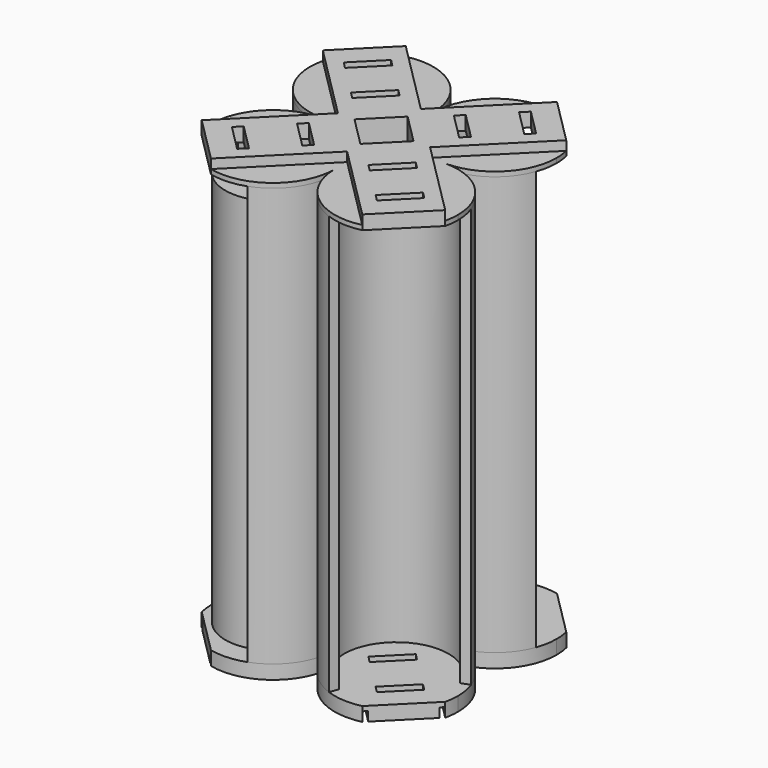
from build123d import *
from build123d import SkipClean  # not in build123d's __all__

# Parameters (mm, degrees)
F1_DEPTH  = 22.5
F2_R      = 5.125
F3_DEPTH  = 43
F4_R      = 1.75
F5_DEPTH  = 2
F6_R      = 5.125
F6_R_2    = 3
F7_DEPTH  = 0.5
F9_DEPTH  = 0.5
F11_DEPTH = 1.5
F13_DEPTH = 1
F14_DEPTH = 47.001
F16_DEPTH = 1


# Not quite as in the source:
# - after a boolean that leaves OpenCascade's solid faulty, fix() repairs it


with BuildPart() as f1:
    # F0 (on Top) → F1 (new body, symmetric)
    with BuildSketch(Plane.XY):
        with BuildLine():
            ThreePointArc((-4.7011366938, 11.9107709919), (-2.0172697509, 9.8513674545), (-1, 6.625))
            ThreePointArc((-1, 6.625), (-5.6482290006, 1.0854563893), (-11.9107709919, 4.7011366938))
            Line((-11.9107709919, 4.7011366938), (-12.8504636127, 4.3591165505))
            ThreePointArc((-12.8504636127, 4.3591165505), (-10.4249438908, 1.1981177066), (-6.625, 0))
            ThreePointArc((-6.625, 0), (-10.4249438908, -1.1981177066), (-12.8504636127, -4.3591165505))
            Line((-12.8504636127, -4.3591165505), (-11.9107709919, -4.7011366938))
            ThreePointArc((-11.9107709919, -4.7011366938), (-5.6482290006, -1.0854563893), (-1, -6.625))
            ThreePointArc((-1, -6.625), (-2.0172697509, -9.8513674545), (-4.7011366938, -11.9107709919))
            Line((-4.7011366938, -11.9107709919), (-4.3591165505, -12.8504636127))
            ThreePointArc((-4.3591165505, -12.8504636127), (-1.1981177066, -10.4249438908), (0, -6.625))
            ThreePointArc((0, -6.625), (1.1981177066, -10.4249438908), (4.3591165505, -12.8504636127))
            Line((4.3591165505, -12.8504636127), (4.7011366938, -11.9107709919))
            ThreePointArc((4.7011366938, -11.9107709919), (2.6475243558, -2.6475243558), (11.9107709919, -4.7011366938))
            Line((11.9107709919, -4.7011366938), (12.8504636127, -4.3591165505))
            ThreePointArc((12.8504636127, -4.3591165505), (10.4249438908, -1.1981177066), (6.625, 0))
            ThreePointArc((6.625, 0), (10.4249438908, 1.1981177066), (12.8504636127, 4.3591165505))
            Line((12.8504636127, 4.3591165505), (11.9107709919, 4.7011366938))
            ThreePointArc((11.9107709919, 4.7011366938), (2.6475243558, 2.6475243558), (4.7011366938, 11.9107709919))
            Line((4.7011366938, 11.9107709919), (4.3591165505, 12.8504636127))
            ThreePointArc((4.3591165505, 12.8504636127), (1.1981177066, 10.4249438908), (0, 6.625))
            ThreePointArc((0, 6.625), (-1.1981177066, 10.4249438908), (-4.3591165505, 12.8504636127))
            Line((-4.3591165505, 12.8504636127), (-4.7011366938, 11.9107709919))
        make_face()
        Polygon((0, -3.1737283681), (-3.1737283681, 0), (0, 3.1737283681), (3.1737283681, 0), align=None, mode=Mode.SUBTRACT)
    extrude(amount=F1_DEPTH, both=True)

    # F8 (on face) → F9 (join)
    with BuildSketch(Plane.XY.offset(22.5)):
        with BuildLine():
            ThreePointArc((-6.625, 0), (-11.3095824254, -11.3095824254), (0, -6.625))
            ThreePointArc((0, -6.625), (-1.9404175746, -1.9404175746), (-6.625, 0))
        make_face()
        Polygon((-10.3373106012, -7.5088834765), (-9.63020382, -6.8017766953), (-6.8017766953, -9.63020382), (-7.5088834765, -10.3373106012), align=None, mode=Mode.SUBTRACT)
        Polygon((-2.9126893988, -5.7411165235), (-3.61979618, -6.4482233047), (-6.4482233047, -3.61979618), (-5.7411165235, -2.9126893988), align=None, mode=Mode.SUBTRACT)
        with BuildLine():
            ThreePointArc((6.6250000363, 0), (1.9404175875, -1.9404175618), (0, -6.625))
            ThreePointArc((0, -6.625), (6.625, -13.25), (13.25, -6.625))
            ThreePointArc((13.25, -6.625), (11.3095824382, -1.9404175875), (6.6250000363, 0))
        make_face()
        Polygon((7.5088834765, -10.3373106012), (6.8017766953, -9.63020382), (9.63020382, -6.8017766953), (10.3373106012, -7.5088834765), align=None, mode=Mode.SUBTRACT)
        Polygon((2.9126893988, -5.7411165235), (5.7411165235, -2.9126893988), (6.4482233047, -3.61979618), (3.61979618, -6.4482233047), align=None, mode=Mode.SUBTRACT)
        with BuildLine():
            ThreePointArc((-6.625, 0), (-1.9404175746, -1.9404175746), (0, -6.625))
            ThreePointArc((0, -6.625), (1.9404175875, -1.9404175618), (6.6250000363, 0))
            ThreePointArc((6.6250000363, 0), (1.9404175875, 1.9404175618), (0, 6.625))
            ThreePointArc((0, 6.625), (-1.9404175746, 1.9404175746), (-6.625, 0))
        make_face()
        Polygon((0, -3.1737283681), (-3.1737283681, 0), (0, 3.1737283681), (3.1737283681, 0), align=None, mode=Mode.SUBTRACT)
        with BuildLine():
            ThreePointArc((0, 6.625), (-11.3095824254, 11.3095824254), (-6.625, 0))
            ThreePointArc((-6.625, 0), (-1.9404175746, 1.9404175746), (0, 6.625))
        make_face()
        Polygon((-2.9126893988, 5.7411165235), (-5.7411165235, 2.9126893988), (-6.4482233047, 3.61979618), (-3.61979618, 6.4482233047), align=None, mode=Mode.SUBTRACT)
        Polygon((-7.5088834765, 10.3373106012), (-6.8017766953, 9.63020382), (-9.63020382, 6.8017766953), (-10.3373106012, 7.5088834765), align=None, mode=Mode.SUBTRACT)
        with BuildLine():
            ThreePointArc((0, 6.625), (1.9404175875, 1.9404175618), (6.6250000363, 0))
            ThreePointArc((6.6250000363, 0), (11.3095824382, 1.9404175875), (13.25, 6.625))
            ThreePointArc((13.25, 6.625), (6.625, 13.25), (0, 6.625))
        make_face()
        Polygon((6.4482233047, 3.61979618), (5.7411165235, 2.9126893988), (2.9126893988, 5.7411165235), (3.61979618, 6.4482233047), align=None, mode=Mode.SUBTRACT)
        Polygon((9.63020382, 6.8017766953), (6.8017766953, 9.63020382), (7.5088834765, 10.3373106012), (10.3373106012, 7.5088834765), align=None, mode=Mode.SUBTRACT)
    with SkipClean():  # cleaning this boolean's faces spoils the solid; the shape is the same uncleaned
        extrude(amount=F9_DEPTH)

    # F10 (on face) → F11 (join)
    with BuildSketch(Plane(origin=(0, 0, -22.5), x_dir=(1, 0, 0), z_dir=(0, 0, -1))):
        with BuildLine():
            ThreePointArc((-6.625, 0), (-11.3095824254, -11.3095824254), (0, -6.625))
            ThreePointArc((0, -6.625), (-1.9404175746, -1.9404175746), (-6.625, 0))
        make_face()
        Polygon((-10.3373106012, -7.5088834765), (-9.63020382, -6.8017766953), (-6.8017766953, -9.63020382), (-7.5088834765, -10.3373106012), align=None, mode=Mode.SUBTRACT)
        Polygon((-2.9126893988, -5.7411165235), (-3.61979618, -6.4482233047), (-6.4482233047, -3.61979618), (-5.7411165235, -2.9126893988), align=None, mode=Mode.SUBTRACT)
        with BuildLine():
            ThreePointArc((6.6250000363, 0), (1.9404175875, -1.9404175618), (0, -6.625))
            ThreePointArc((0, -6.625), (6.625, -13.25), (13.25, -6.625))
            ThreePointArc((13.25, -6.625), (11.3095824382, -1.9404175875), (6.6250000363, 0))
        make_face()
        Polygon((7.5088834765, -10.3373106012), (6.8017766953, -9.63020382), (9.63020382, -6.8017766953), (10.3373106012, -7.5088834765), align=None, mode=Mode.SUBTRACT)
        Polygon((2.9126893988, -5.7411165235), (5.7411165235, -2.9126893988), (6.4482233047, -3.61979618), (3.61979618, -6.4482233047), align=None, mode=Mode.SUBTRACT)
        with BuildLine():
            ThreePointArc((-6.625, 0), (-1.9404175746, -1.9404175746), (0, -6.625))
            ThreePointArc((0, -6.625), (1.9404175875, -1.9404175618), (6.6250000363, 0))
            ThreePointArc((6.6250000363, 0), (1.9404175875, 1.9404175618), (0, 6.625))
            ThreePointArc((0, 6.625), (-1.9404175746, 1.9404175746), (-6.625, 0))
        make_face()
        Polygon((0, -3.1737283681), (-3.1737283681, 0), (0, 3.1737283681), (3.1737283681, 0), align=None, mode=Mode.SUBTRACT)
        with BuildLine():
            ThreePointArc((0, 6.625), (-11.3095824254, 11.3095824254), (-6.625, 0))
            ThreePointArc((-6.625, 0), (-1.9404175746, 1.9404175746), (0, 6.625))
        make_face()
        Polygon((-2.9126893988, 5.7411165235), (-5.7411165235, 2.9126893988), (-6.4482233047, 3.61979618), (-3.61979618, 6.4482233047), align=None, mode=Mode.SUBTRACT)
        Polygon((-7.5088834765, 10.3373106012), (-6.8017766953, 9.63020382), (-9.63020382, 6.8017766953), (-10.3373106012, 7.5088834765), align=None, mode=Mode.SUBTRACT)
        with BuildLine():
            ThreePointArc((0, 6.625), (1.9404175875, 1.9404175618), (6.6250000363, 0))
            ThreePointArc((6.6250000363, 0), (11.3095824382, 1.9404175875), (13.25, 6.625))
            ThreePointArc((13.25, 6.625), (6.625, 13.25), (0, 6.625))
        make_face()
        Polygon((6.4482233047, 3.61979618), (5.7411165235, 2.9126893988), (2.9126893988, 5.7411165235), (3.61979618, 6.4482233047), align=None, mode=Mode.SUBTRACT)
        Polygon((9.63020382, 6.8017766953), (6.8017766953, 9.63020382), (7.5088834765, 10.3373106012), (10.3373106012, 7.5088834765), align=None, mode=Mode.SUBTRACT)
    with SkipClean():  # cleaning this boolean's faces spoils the solid; the shape is the same uncleaned
        extrude(amount=F11_DEPTH)

    # F12 (on face) → F13 (join)
    with BuildSketch(Plane.XY.offset(23)):
        Polygon((8.12760191, 13.0773493783), (0, 4.9497474683), (-8.12760191, 13.0773493783), (-13.0773493783, 8.12760191), (-4.9497474683, 0), (-13.0773493783, -8.12760191), (-8.12760191, -13.0773493783), (0, -4.9497474683), (8.12760191, -13.0773493783), (13.0773493783, -8.12760191), (4.9497474683, 0), (13.0773493783, 8.12760191), align=None)
        Polygon((-9.63020382, -6.8017766953), (-6.8017766953, -9.63020382), (-7.5088834765, -10.3373106012), (-10.3373106012, -7.5088834765), align=None, mode=Mode.SUBTRACT)
        Polygon((-5.7411165235, -2.9126893988), (-2.9126893988, -5.7411165235), (-3.61979618, -6.4482233047), (-6.4482233047, -3.61979618), align=None, mode=Mode.SUBTRACT)
        Polygon((7.5088834765, -10.3373106012), (6.8017766953, -9.63020382), (9.63020382, -6.8017766953), (10.3373106012, -7.5088834765), align=None, mode=Mode.SUBTRACT)
        Polygon((3.61979618, -6.4482233047), (2.9126893988, -5.7411165235), (5.7411165235, -2.9126893988), (6.4482233047, -3.61979618), align=None, mode=Mode.SUBTRACT)
        Polygon((-5.7411165235, 2.9126893988), (-6.4482233047, 3.61979618), (-3.61979618, 6.4482233047), (-2.9126893988, 5.7411165235), align=None, mode=Mode.SUBTRACT)
        Polygon((-9.63020382, 6.8017766953), (-10.3373106012, 7.5088834765), (-7.5088834765, 10.3373106012), (-6.8017766953, 9.63020382), align=None, mode=Mode.SUBTRACT)
        Polygon((0, -3.1737283681), (-3.1737283681, 0), (0, 3.1737283681), (3.1737283681, 0), align=None, mode=Mode.SUBTRACT)
        Polygon((2.9126893988, 5.7411165235), (3.61979618, 6.4482233047), (6.4482233047, 3.61979618), (5.7411165235, 2.9126893988), align=None, mode=Mode.SUBTRACT)
        Polygon((10.3373106012, 7.5088834765), (9.63020382, 6.8017766953), (6.8017766953, 9.63020382), (7.5088834765, 10.3373106012), align=None, mode=Mode.SUBTRACT)
    extrude(amount=F13_DEPTH)

    add(f1.part.fix(), mode=Mode.REPLACE)

    # F14 (cut, through all): faces of the model
    f14_faces = [f1.faces().sort_by_distance(p)[0] for p in [
        (10.8872317954, -10.8872317954, 23),
        (-10.8872317954, -10.8872317954, 23),
        (-10.8872317954, 10.8872317954, 23),
        (10.8872317954, 10.8872317954, 23),
    ]]
    extrude(f14_faces, amount=-F14_DEPTH, mode=Mode.SUBTRACT)

    # F15 (on face) → F16 (cut)
    with BuildSketch(Plane(origin=(0, 0, -24), x_dir=(1, 0, 0), z_dir=(0, 0, -1))):
        Polygon((-5.6527281759, 1.4100874887), (-12.7237959877, 8.4811553006), (-13.0773493783, 8.12760191), (-6.0062815665, 1.0565340982), align=None)
        Polygon((-8.12760191, 13.0773493783), (-8.4811553006, 12.7237959877), (-1.4100874887, 5.6527281759), (-1.0565340982, 6.0062815665), align=None)
        Polygon((8.12760191, 13.0773493783), (1.0565340982, 6.0062815665), (1.4100874887, 5.6527281759), (8.4811553006, 12.7237959877), align=None)
        Polygon((13.0773493783, 8.12760191), (12.7237959877, 8.4811553006), (5.6527281759, 1.4100874887), (6.0062815665, 1.0565340982), align=None)
        Polygon((-5.6527281759, -1.4100874887), (-6.0062815665, -1.0565340982), (-13.0773493783, -8.12760191), (-12.7237959877, -8.4811553006), align=None)
        Polygon((-1.4100874887, -5.6527281759), (-8.4811553006, -12.7237959877), (-8.12760191, -13.0773493783), (-1.0565340982, -6.0062815665), align=None)
        Polygon((1.4100874887, -5.6527281759), (1.0565340982, -6.0062815665), (8.12760191, -13.0773493783), (8.4811553006, -12.7237959877), align=None)
        Polygon((5.6527281759, -1.4100874887), (12.7237959877, -8.4811553006), (13.0773493783, -8.12760191), (6.0062815665, -1.0565340982), align=None)
    extrude(amount=-F16_DEPTH, mode=Mode.SUBTRACT)


with BuildPart() as f3:
    # F2 (on face) → F3 (new body)
    with BuildSketch(Plane(origin=(0, 0, -22.5), x_dir=(1, 0, 0), z_dir=(0, 0, -1))):
        with Locations((-6.625, 6.625)):
            Circle(F2_R)
    extrude(amount=-F3_DEPTH)

    # F4 (on face) → F5 (join)
    with BuildSketch(Plane.XY.offset(20.5)):
        with Locations((-6.625, -6.625)):
            Circle(F4_R)
    extrude(amount=F5_DEPTH)

    # F6 (on face) → F7 (cut)
    with BuildSketch(Plane(origin=(0, 0, -22.5), x_dir=(1, 0, 0), z_dir=(0, 0, -1))):
        with Locations((-6.625, 6.625)):
            Circle(F6_R)
        with Locations((-6.625, 6.625)):
            Circle(F6_R_2, mode=Mode.SUBTRACT)
    extrude(amount=-F7_DEPTH, mode=Mode.SUBTRACT)


solid = Compound([f1.part, f3.part])
